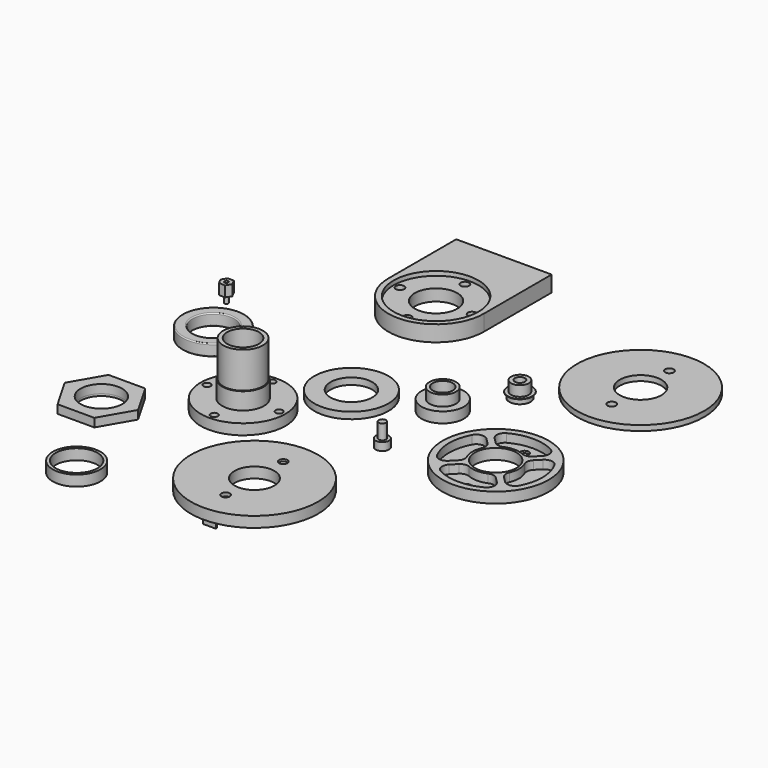
from build123d import *
from build123d import SkipClean  # not in build123d's __all__

# Parameters (mm, degrees)
F0_R      = 25.4
F1_DEPTH  = 6.35
F2_R      = 12.4968
F3_DEPTH  = 10.16
F4_R      = 11.90625
F5_DEPTH  = 21.59
F6_R      = 9.525
F7_DEPTH  = 38.101
F8_R      = 2.159
F9_DEPTH  = 38.101
F10_R     = 22.225
F10_R_2   = 12.4968
F11_DEPTH = 3.9878
F12_R     = 18.5039
F12_R_2   = 12.4968
F13_DEPTH = 7.0104
F14_R     = 0.635
F16_DEPTH = 5.08
F17_R     = 12.4968
F18_DEPTH = 38.101
F19_R     = 13.335
F19_R_2   = 12.4968
F20_DEPTH = 1.27
F21_R     = 38.1
F21_R_2   = 11.90625
F22_DEPTH = 6.35
F23_R     = 12.7
F24_DEPTH = 6.35
F25_R     = 7.9375
F26_DEPTH = 6.35
F27_R     = 14.2875
F27_R_2   = 12.4968
F28_DEPTH = 6.35
F29_R     = 5.9944
F30_DEPTH = 13.971
F32_DEPTH = 9.525
F33_R     = 25.4
F33_R_2   = 12.7
F34_DEPTH = 2.54
F35_R     = 2.54
F36_DEPTH = 8.256
F37_R     = 2.159
F38_DEPTH = 12.7
F39_R     = 4.0005
F40_DEPTH = 4.699
F41_R     = 2.159
F42_DEPTH = 8.89
F43_R     = 2.54
F44_DEPTH = 7.621
F45_R     = 2.54
F46_DEPTH = 5.08
F47_R     = 13.6525
F48_DEPTH = 0.508
F49_R     = 31.75
F49_R_2   = 12.4968
F50_DEPTH = 6.35
F52_DEPTH = 5.08
F53_R     = 2.54
F54_DEPTH = 38.101
F55_R     = 6.35
F56_DEPTH = 3.175
F57_R     = 5.334
F58_DEPTH = 6.35
F59_R     = 3
F60_DEPTH = 10.796
F61_R     = 38.1
F61_R_2   = 2.54
F61_R_3   = 12.5
F62_DEPTH = 3.175
F64_DEPTH = 6.35
F65_R     = 1.1303
F66_DEPTH = 4.7625
F67_R     = 1.1303
F68_DEPTH = 4.7625
F69_R     = 7.4295
F69_R_2   = 3.81
F70_DEPTH = 0.254
F71_W     = 7.62
F71_H     = 13.97
F71_R     = 2.54
F72_DEPTH = 0.889
F73_W     = 7.62
F73_H     = 0.889
F74_DEPTH = 6.35
F75_W     = 7.62
F75_H     = 0.889
F76_DEPTH = 1.905
F77_W     = 7.62
F77_H     = 0.889
F78_DEPTH = 3.175


with BuildPart() as f1:
    # F0 (on Top) → F1 (new body)
    with BuildSketch(Plane.XY):
        Circle(F0_R)
    extrude(amount=F1_DEPTH)

    # F2 (on face) → F3 (join)
    with BuildSketch(Plane.XY.offset(6.35)):
        Circle(F2_R)
    extrude(amount=F3_DEPTH)

    # F4 (on face) → F5 (join)
    with BuildSketch(Plane.XY.offset(16.51)):
        Circle(F4_R)
    extrude(amount=F5_DEPTH)

    # F6 (on face) → F7 (cut, through all)
    with BuildSketch(Plane(origin=(0, 0, 0), x_dir=(1, 0, 0), z_dir=(0, 0, -1))):
        Circle(F6_R)
    extrude(amount=-F7_DEPTH, mode=Mode.SUBTRACT)

    # F8 (on face) → F9 (cut, through all)
    with BuildSketch(Plane(origin=(0, 0, 0), x_dir=(1, 0, 0), z_dir=(0, 0, -1))):
        with Locations((0, -21.59)):
            Circle(F8_R)
        with Locations((21.59, 0)):
            Circle(F8_R)
        with Locations((-21.59, 0)):
            Circle(F8_R)
        with Locations((0, 21.59)):
            Circle(F8_R)
    extrude(amount=-F9_DEPTH, mode=Mode.SUBTRACT)


with BuildPart() as f11:
    # F10 (on Top) → F11 (new body)
    with BuildSketch(Plane.XY):
        with Locations((31.3683748245, 41.8724641204)):
            Circle(F10_R)
        with Locations((31.3683748245, 41.8724641204)):
            Circle(F10_R_2, mode=Mode.SUBTRACT)
    extrude(amount=F11_DEPTH)


with BuildPart() as f13:
    # F12 (on Top) → F13 (new body)
    with BuildSketch(Plane.XY):
        with Locations((-56.1177358031, 47.9159131646)):
            Circle(F12_R)
        with Locations((-56.1177358031, 47.9159131646)):
            Circle(F12_R_2, mode=Mode.SUBTRACT)
    extrude(amount=F13_DEPTH)

    # F14
    f14_edges = [f13.edges().sort_by_distance(p)[0] for p in [
        (-74.621636, 47.915913, 7.0104),
        (-68.614536, 47.915913, 7.0104),
        (-43.620936, 47.915913, 3.5052),
        (-68.614536, 47.915913, 0),
        (-37.613836, 47.915913, 3.5052),
        (-74.621636, 47.915913, 0),
    ]]
    fillet(f14_edges, radius=F14_R)


with BuildPart() as f16:
    # F15 (on Top) → F16 (new body)
    with BuildSketch(Plane.XY):
        Polygon((-65.4306539781, -18.943020756), (-76.4291766062, -37.993020756), (-65.4306539781, -57.043020756), (-43.433608722, -57.043020756), (-32.4350860939, -37.993020756), (-43.433608722, -18.943020756), align=None)
    extrude(amount=F16_DEPTH)

    # F17 (on face) → F18 (cut, through all)
    with BuildSketch(Plane(origin=(0, 0, 0), x_dir=(1, 0, 0), z_dir=(0, 0, -1))):
        with Locations((-54.43213135, 37.993020756)):
            Circle(F17_R)
    extrude(amount=-F18_DEPTH, mode=Mode.SUBTRACT)

    # F19 (on face) → F20 (join)
    with BuildSketch(Plane(origin=(0, 0, 0), x_dir=(1, 0, 0), z_dir=(0, 0, -1))):
        with Locations((-54.43213135, 37.993020756)):
            Circle(F19_R)
        with Locations((-54.43213135, 37.993020756)):
            Circle(F19_R_2, mode=Mode.SUBTRACT)
    extrude(amount=F20_DEPTH)


with BuildPart() as f22:
    # F21 (on Top) → F22 (new body)
    with BuildSketch(Plane.XY):
        with Locations((54.7905638814, -59.9489323795)):
            Circle(F21_R)
        with Locations((54.7905638814, -59.9489323795)):
            Circle(F21_R_2, mode=Mode.SUBTRACT)
    extrude(amount=F22_DEPTH)

    # F43 (on face) → F44 (cut, through all)
    with BuildSketch(Plane.XY.offset(6.35)):
        with Locations((54.7905638814, -81.5389323795)):
            Circle(F43_R)
        with Locations((54.7905638814, -38.3589323795)):
            Circle(F43_R)
    extrude(amount=-F44_DEPTH, mode=Mode.SUBTRACT)

    # F45 (on face) → F46 (cut)
    with BuildSketch(Plane(origin=(0, 0, 0), x_dir=(1, 0, 0), z_dir=(0, 0, -1))):
        Polygon((57.4846407177, 59.9489323795), (54.7905638814, 62.6430092158), (52.0964870451, 59.9489323795), (54.7905638814, 57.2548555432), align=None)
        with BuildLine():
            Line((45.4458163169, 47.9101079786), (32.827825649, 35.2921173107))
            ThreePointArc((32.827825649, 35.2921173107), (54.7905638814, 26.9289323795), (76.7533021138, 35.2921173107))
            Line((76.7533021138, 35.2921173107), (64.1353114459, 47.9101079786))
            ThreePointArc((64.1353114459, 47.9101079786), (54.7905638814, 44.7089323795), (45.4458163169, 47.9101079786))
        make_face()
        with Locations((54.7905638814, 38.3589323795)):
            Circle(F45_R, mode=Mode.SUBTRACT)
        with BuildLine():
            Line((79.4473789501, 81.9116706119), (66.8293882823, 69.293679944))
            ThreePointArc((66.8293882823, 69.293679944), (70.0305638814, 59.9489323795), (66.8293882823, 50.6041848149))
            Line((66.8293882823, 50.6041848149), (79.4473789501, 37.9861941471))
            ThreePointArc((79.4473789501, 37.9861941471), (87.8105638814, 59.9489323795), (79.4473789501, 81.9116706119))
        make_face()
        with BuildLine():
            ThreePointArc((76.7533021138, 84.6057474482), (54.7905638814, 92.9689323795), (32.827825649, 84.6057474482))
            Line((32.827825649, 84.6057474482), (45.4458163169, 71.9877567804))
            ThreePointArc((45.4458163169, 71.9877567804), (54.7905638814, 75.1889323795), (64.1353114459, 71.9877567804))
            Line((64.1353114459, 71.9877567804), (76.7533021138, 84.6057474482))
        make_face()
        with Locations((54.7905638814, 81.5389323795)):
            Circle(F45_R, mode=Mode.SUBTRACT)
        with BuildLine():
            Line((42.7517394805, 69.293679944), (30.1337488127, 81.9116706119))
            ThreePointArc((30.1337488127, 81.9116706119), (21.7705638814, 59.9489323795), (30.1337488127, 37.9861941471))
            Line((30.1337488127, 37.9861941471), (42.7517394805, 50.6041848149))
            ThreePointArc((42.7517394805, 50.6041848149), (39.5505638814, 59.9489323795), (42.7517394805, 69.293679944))
        make_face()
    extrude(amount=-F46_DEPTH, mode=Mode.SUBTRACT)

    # F47 (on face) → F48 (cut)
    with BuildSketch(Plane(origin=(0, 0, 0), x_dir=(1, 0, 0), z_dir=(0, 0, -1))):
        with BuildLine():
            Line((42.7517394805, 69.293679944), (30.1337488127, 81.9116706119))
            ThreePointArc((30.1337488127, 81.9116706119), (21.7705638814, 59.9489323795), (30.1337488127, 37.9861941471))
            Line((30.1337488127, 37.9861941471), (42.7517394805, 50.6041848149))
            ThreePointArc((42.7517394805, 50.6041848149), (39.5505638814, 59.9489323795), (42.7517394805, 69.293679944))
        make_face()
        with BuildLine():
            ThreePointArc((79.4473789501, 37.9861941471), (85.6490184244, 48.1983501294), (87.8105638814, 59.9489323795))
            ThreePointArc((87.8105638814, 59.9489323795), (85.6490184244, 71.6995146295), (79.4473789501, 81.9116706119))
            Line((79.4473789501, 81.9116706119), (66.8293882823, 69.293679944))
            ThreePointArc((66.8293882823, 69.293679944), (70.0305638814, 59.9489323795), (66.8293882823, 50.6041848149))
            Line((66.8293882823, 50.6041848149), (79.4473789501, 37.9861941471))
        make_face()
        with BuildLine():
            ThreePointArc((32.827825649, 35.2921173107), (54.7905638814, 26.9289323795), (76.7533021138, 35.2921173107))
            Line((76.7533021138, 35.2921173107), (64.1353114459, 47.9101079786))
            ThreePointArc((64.1353114459, 47.9101079786), (54.7905638814, 44.7089323795), (45.4458163169, 47.9101079786))
            Line((45.4458163169, 47.9101079786), (32.827825649, 35.2921173107))
        make_face()
        with BuildLine():
            Line((64.1353114459, 71.9877567804), (76.7533021138, 84.6057474482))
            ThreePointArc((76.7533021138, 84.6057474482), (54.7905638814, 92.9689323795), (32.827825649, 84.6057474482))
            Line((32.827825649, 84.6057474482), (45.4458163169, 71.9877567804))
            ThreePointArc((45.4458163169, 71.9877567804), (54.7905638814, 75.1889323795), (64.1353114459, 71.9877567804))
        make_face()
        with BuildLine():
            Line((66.8293882823, 69.293679944), (79.4473789501, 81.9116706119))
            ThreePointArc((79.4473789501, 81.9116706119), (78.1392297962, 83.2975982943), (76.7533021138, 84.6057474482))
            Line((76.7533021138, 84.6057474482), (64.1353114459, 71.9877567804))
            ThreePointArc((64.1353114459, 71.9877567804), (54.7905638814, 75.1889323795), (45.4458163169, 71.9877567804))
            Line((45.4458163169, 71.9877567804), (32.827825649, 84.6057474482))
            ThreePointArc((32.827825649, 84.6057474482), (31.4418979666, 83.2975982943), (30.1337488127, 81.9116706119))
            Line((30.1337488127, 81.9116706119), (42.7517394805, 69.293679944))
            ThreePointArc((42.7517394805, 69.293679944), (39.5505638814, 59.9489323795), (42.7517394805, 50.6041848149))
            Line((42.7517394805, 50.6041848149), (30.1337488127, 37.9861941471))
            ThreePointArc((30.1337488127, 37.9861941471), (31.4418979666, 36.6002664647), (32.827825649, 35.2921173107))
            Line((32.827825649, 35.2921173107), (45.4458163169, 47.9101079786))
            ThreePointArc((45.4458163169, 47.9101079786), (54.7905638814, 44.7089323795), (64.1353114459, 47.9101079786))
            Line((64.1353114459, 47.9101079786), (76.7533021138, 35.2921173107))
            ThreePointArc((76.7533021138, 35.2921173107), (78.1392297962, 36.6002664647), (79.4473789501, 37.9861941471))
            Line((79.4473789501, 37.9861941471), (66.8293882823, 50.6041848149))
            ThreePointArc((66.8293882823, 50.6041848149), (70.0305638814, 59.9489323795), (66.8293882823, 69.293679944))
        make_face()
        with Locations((54.7905638814, 59.9489323795)):
            Circle(F47_R, mode=Mode.SUBTRACT)
    with SkipClean():  # cleaning this boolean's faces spoils the solid; the shape is the same uncleaned
        extrude(amount=-F48_DEPTH, mode=Mode.SUBTRACT)


with BuildPart() as f24:
    # F23 (on Top) → F24 (new body)
    with BuildSketch(Plane.XY):
        with Locations((73.2964575291, 57.8182339668)):
            Circle(F23_R)
    extrude(amount=F24_DEPTH)

    # F25 (on face) → F26 (join)
    with BuildSketch(Plane.XY.offset(6.35)):
        with Locations((73.2964575291, 57.8182339668)):
            Circle(F25_R)
    extrude(amount=F26_DEPTH)

    # F29 (on face) → F30 (cut, through all)
    with BuildSketch(Plane.XY.offset(12.7)):
        with Locations((73.2964575291, 57.8182339668)):
            Circle(F29_R)
    extrude(amount=-F30_DEPTH, mode=Mode.SUBTRACT)


with BuildPart() as f28:
    # F27 (on Top) → F28 (new body)
    with BuildSketch(Plane.XY):
        with Locations((-21.3446542621, -97.8919789195)):
            Circle(F27_R)
        with Locations((-21.3446542621, -97.8919789195)):
            Circle(F27_R_2, mode=Mode.SUBTRACT)
    extrude(amount=F28_DEPTH)


with BuildPart() as f32:
    # F31 (on Top) → F32 (new body)
    with BuildSketch(Plane.XY):
        with BuildLine():
            ThreePointArc((-18.9220272005, 132.3840916157), (9.6529727995, 160.9590916157), (38.2279727995, 132.3840916157))
            Line((38.2279727995, 132.3840916157), (38.2279727995, 183.1840916157))
            Line((38.2279727995, 183.1840916157), (-18.9220272005, 183.1840916157))
            Line((-18.9220272005, 183.1840916157), (-18.9220272005, 132.3840916157))
        make_face()
        with BuildLine():
            ThreePointArc((-18.9220272005, 132.3840916157), (9.6529727995, 103.8090916157), (38.2279727995, 132.3840916157))
            Line((38.2279727995, 132.3840916157), (22.3529727995, 132.3840916157))
            ThreePointArc((22.3529727995, 132.3840916157), (9.6529727995, 119.6840916157), (-3.0470272005, 132.3840916157))
            Line((-3.0470272005, 132.3840916157), (-18.9220272005, 132.3840916157))
        make_face()
        with BuildLine():
            Line((22.3529727995, 132.3840916157), (38.2279727995, 132.3840916157))
            ThreePointArc((38.2279727995, 132.3840916157), (9.6529727995, 160.9590916157), (-18.9220272005, 132.3840916157))
            Line((-18.9220272005, 132.3840916157), (-3.0470272005, 132.3840916157))
            ThreePointArc((-3.0470272005, 132.3840916157), (9.6529727995, 145.0840916157), (22.3529727995, 132.3840916157))
        make_face()
    extrude(amount=F32_DEPTH)

    # F33 (on face) → F34 (cut)
    with BuildSketch(Plane.XY.offset(9.525)):
        with Locations((9.6529727995, 132.3840916157)):
            Circle(F33_R)
        with Locations((9.6529727995, 132.3840916157)):
            Circle(F33_R_2, mode=Mode.SUBTRACT)
    extrude(amount=-F34_DEPTH, mode=Mode.SUBTRACT)

    # F35 (on face) → F36 (cut, through all)
    with BuildSketch(Plane.XY.offset(6.985)):
        with Locations((9.6529727995, 153.9740916157)):
            Circle(F35_R)
        with Locations((31.2429727995, 132.3840916157)):
            Circle(F35_R)
        with Locations((9.6529727995, 110.7940916157)):
            Circle(F35_R)
        with Locations((-11.9370272005, 132.3840916157)):
            Circle(F35_R)
    extrude(amount=-F36_DEPTH, mode=Mode.SUBTRACT)

    # F37 (on face) → F38 (cut)
    with BuildSketch(Plane(origin=(0, 183.1840916157, 0), x_dir=(-1, 0, 0), z_dir=(0, 1, 0))):
        with Locations((14.1595272005, 4.7625)):
            Circle(F37_R)
        with Locations((-33.4654727995, 4.7625)):
            Circle(F37_R)
    extrude(amount=-F38_DEPTH, mode=Mode.SUBTRACT)


with BuildPart() as f40:
    # F39 (on Top) → F40 (new body)
    with BuildSketch(Plane.XY):
        with Locations((74.1678923368, 11.5195177495)):
            Circle(F39_R)
    extrude(amount=F40_DEPTH)

    # F41 (on face) → F42 (join)
    with BuildSketch(Plane.XY.offset(4.699)):
        with Locations((74.1678923368, 11.5195177495)):
            Circle(F41_R)
    extrude(amount=F42_DEPTH)


with BuildPart() as f50:
    # F49 (on Top) → F50 (new body)
    with BuildSketch(Plane.XY):
        with Locations((131.4873993397, 24.7538406402)):
            Circle(F49_R)
        with Locations((131.4873993397, 24.7538406402)):
            Circle(F49_R_2, mode=Mode.SUBTRACT)
    extrude(amount=F50_DEPTH)

    # F51 (on face) → F52 (cut)
    with BuildSketch(Plane.XY.offset(6.35)):
        with BuildLine():
            ThreePointArc((114.5046544296, 39.0425087139), (110.381730574, 40.4034347031), (106.8338098236, 37.9008602253))
            ThreePointArc((106.8338098236, 37.9008602253), (103.5473993397, 24.7538406402), (106.8338098236, 11.606821055))
            ThreePointArc((106.8338098236, 11.606821055), (110.381730574, 9.1042465773), (114.5046544296, 10.4651725665))
            Line((114.5046544296, 10.4651725665), (117.7310246177, 13.6915427546))
            ThreePointArc((117.7310246177, 13.6915427546), (119.0638378135, 16.2252317668), (118.7267511959, 19.0681780621))
            ThreePointArc((118.7267511959, 19.0681780621), (117.5173993397, 24.7538406402), (118.7267511959, 30.4395032183))
            ThreePointArc((118.7267511959, 30.4395032183), (119.0638378135, 33.2824495135), (117.7310246177, 35.8161385258))
            Line((117.7310246177, 35.8161385258), (114.5046544296, 39.0425087139))
        make_face()
        with BuildLine():
            Line((120.4251014541, 10.9974659183), (117.198731266, 7.7710957302))
            ThreePointArc((117.198731266, 7.7710957302), (115.8378052768, 3.6481718745), (118.3403797545, 0.1002511241))
            ThreePointArc((118.3403797545, 0.1002511241), (131.4873993397, -3.1861593598), (144.6344189248, 0.1002511241))
            ThreePointArc((144.6344189248, 0.1002511241), (147.1369934026, 3.6481718745), (145.7760674134, 7.7710957302))
            Line((145.7760674134, 7.7710957302), (142.5496972253, 10.9974659183))
            ThreePointArc((142.5496972253, 10.9974659183), (140.016008213, 12.330279114), (137.1730619178, 11.9931924965))
            ThreePointArc((137.1730619178, 11.9931924965), (131.4873993397, 10.7838406402), (125.8017367616, 11.9931924965))
            ThreePointArc((125.8017367616, 11.9931924965), (122.9587904663, 12.330279114), (120.4251014541, 10.9974659183))
        make_face()
        with BuildLine():
            ThreePointArc((118.3403797545, 49.4074301563), (115.8378052768, 45.8595094059), (117.198731266, 41.7365855502))
            Line((117.198731266, 41.7365855502), (120.4251014541, 38.5102153621))
            ThreePointArc((120.4251014541, 38.5102153621), (122.9587904663, 37.1774021664), (125.8017367616, 37.5144887839))
            ThreePointArc((125.8017367616, 37.5144887839), (131.4873993397, 38.7238406402), (137.1730619178, 37.5144887839))
            ThreePointArc((137.1730619178, 37.5144887839), (140.016008213, 37.1774021664), (142.5496972253, 38.5102153621))
            Line((142.5496972253, 38.5102153621), (145.7760674134, 41.7365855502))
            ThreePointArc((145.7760674134, 41.7365855502), (147.1369934026, 45.8595094059), (144.6344189248, 49.4074301563))
            ThreePointArc((144.6344189248, 49.4074301563), (131.4873993397, 52.6938406402), (118.3403797545, 49.4074301563))
        make_face()
        with BuildLine():
            ThreePointArc((148.4701442497, 10.4651725665), (152.5930681054, 9.1042465773), (156.1409888558, 11.606821055))
            ThreePointArc((156.1409888558, 11.606821055), (159.4273993397, 24.7538406402), (156.1409888558, 37.9008602253))
            ThreePointArc((156.1409888558, 37.9008602253), (152.5930681054, 40.4034347031), (148.4701442497, 39.0425087139))
            Line((148.4701442497, 39.0425087139), (145.2437740616, 35.8161385258))
            ThreePointArc((145.2437740616, 35.8161385258), (143.9109608659, 33.2824495135), (144.2480474834, 30.4395032183))
            ThreePointArc((144.2480474834, 30.4395032183), (145.4573993397, 24.7538406402), (144.2480474834, 19.0681780621))
            ThreePointArc((144.2480474834, 19.0681780621), (143.9109608659, 16.2252317668), (145.2437740616, 13.6915427546))
            Line((145.2437740616, 13.6915427546), (148.4701442497, 10.4651725665))
        make_face()
    extrude(amount=-F52_DEPTH, mode=Mode.SUBTRACT)

    # F53 (on face) → F54 (cut, through all)
    with BuildSketch(Plane(origin=(0, 0, 0), x_dir=(1, 0, 0), z_dir=(0, 0, -1))):
        with Locations((131.4873993397, -46.3438406402)):
            Circle(F53_R)
        with Locations((131.4873993397, -3.1638406402)):
            Circle(F53_R)
    extrude(amount=-F54_DEPTH, mode=Mode.SUBTRACT)


with BuildPart() as f56:
    # F55 (on Top) → F56 (new body)
    with BuildSketch(Plane.XY):
        with Locations((93.3464094996, 90.5423536897)):
            Circle(F55_R)
    extrude(amount=F56_DEPTH)

    # F57 (on face) → F58 (join)
    with BuildSketch(Plane.XY.offset(3.175)):
        with Locations((93.3464094996, 90.5423536897)):
            Circle(F57_R)
    extrude(amount=F58_DEPTH)

    # F59 (on face) → F60 (cut, through all)
    with BuildSketch(Plane.XY.offset(9.525)):
        with Locations((93.3464094996, 90.5423536897)):
            Circle(F59_R)
    extrude(amount=-F60_DEPTH, mode=Mode.SUBTRACT)

    # F69 (on face) → F70 (join)
    with BuildSketch(Plane.XY.offset(3.175)):
        with Locations((93.3464094996, 90.5423536897)):
            Circle(F69_R)
        with Locations((93.3464094996, 90.5423536897)):
            Circle(F69_R_2, mode=Mode.SUBTRACT)
    extrude(amount=F70_DEPTH)


with BuildPart() as f62:
    # F61 (on Top) → F62 (new body)
    with BuildSketch(Plane.XY):
        with Locations((134.5105986134, 129.3833033046)):
            Circle(F61_R)
        with Locations((134.5105986134, 107.7933033046)):
            Circle(F61_R_2, mode=Mode.SUBTRACT)
        with Locations((134.5105986134, 129.3833033046)):
            Circle(F61_R_3, mode=Mode.SUBTRACT)
        with Locations((134.5105986134, 150.9733033046)):
            Circle(F61_R_2, mode=Mode.SUBTRACT)
    extrude(amount=F62_DEPTH)


with BuildPart() as f64:
    # F63 (on Top) → F64 (new body)
    with BuildSketch(Plane.XY):
        Polygon((-78.0116962825, 83.9019809232), (-76.0501052281, 86.9992367842), (-77.7516119585, 90.2466523997), (-81.4147097434, 90.3968121542), (-83.3763007978, 87.2995562932), (-81.6747940674, 84.0521406777), align=None)
    extrude(amount=F64_DEPTH)

    # F65 (on face) → F66 (cut)
    with BuildSketch(Plane.XY.offset(6.35)):
        with Locations((-79.7132030129, 87.1493965387)):
            Circle(F65_R)
    extrude(amount=-F66_DEPTH, mode=Mode.SUBTRACT)

    # F67 (on face) → F68 (join)
    with BuildSketch(Plane(origin=(0, 0, 0), x_dir=(1, 0, 0), z_dir=(0, 0, -1))):
        with Locations((-79.7132030129, -87.1493965387)):
            Circle(F67_R)
    extrude(amount=F68_DEPTH)


with BuildPart() as f72:
    # F71 (on face) → F72 (new body)
    with BuildSketch(Plane(origin=(0, 0, 5.08), x_dir=(1, 0, 0), z_dir=(0, 0, -1))):
        with Locations((54.7905638814, 84.7139323795)):
            Rectangle(F71_W, F71_H)
        with Locations((54.7905638814, 81.5389323795)):
            Circle(F71_R, mode=Mode.SUBTRACT)
    extrude(amount=F72_DEPTH)

    # F73 (on face) → F74 (join)
    with BuildSketch(Plane(origin=(0, 0, 4.191), x_dir=(1, 0, 0), z_dir=(0, 0, -1))):
        with Locations((54.7905638814, 91.2544323795)):
            Rectangle(F73_W, F73_H)
    extrude(amount=F74_DEPTH)

    # F75 (on face) → F76 (join)
    with BuildSketch(Plane.XZ.offset(91.6989323795)):
        with Locations((54.7905638814, -1.7145)):
            Rectangle(F75_W, F75_H)
    extrude(amount=F76_DEPTH)

    # F77 (on face) → F78 (join)
    with BuildSketch(Plane(origin=(0, 0, -2.159), x_dir=(1, 0, 0), z_dir=(0, 0, -1))):
        with Locations((54.7905638814, 93.1594323795)):
            Rectangle(F77_W, F77_H)
    extrude(amount=F78_DEPTH)


solid = Compound([f1.part, f11.part, f13.part, f16.part, f22.part, f24.part, f28.part, f32.part, f40.part, f50.part, f56.part, f62.part, f64.part, f72.part])
